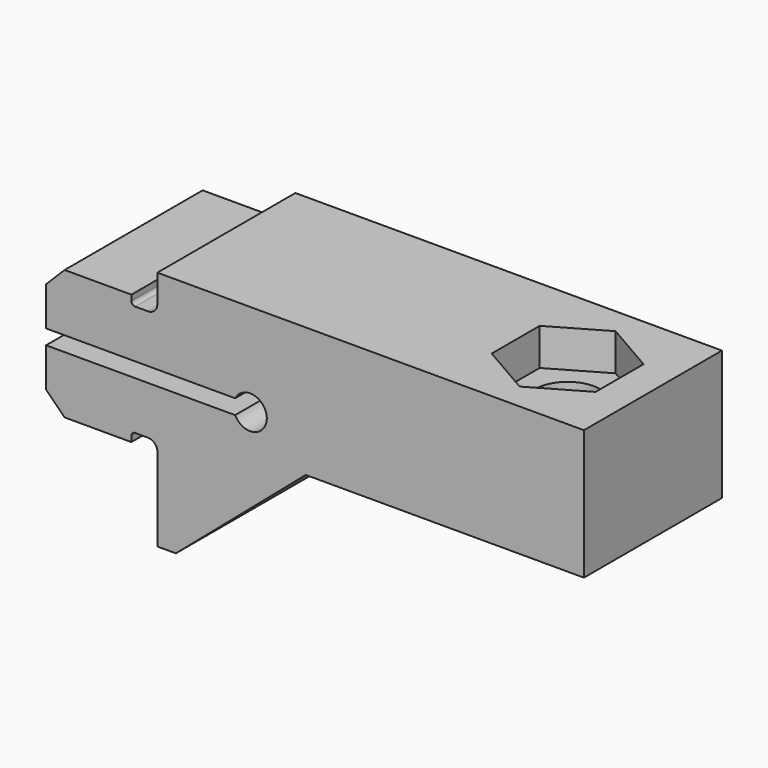
from build123d import *

# Parameters (mm, degrees)
F1_DEPTH = 4.65
F2_R     = 1.75
F3_DEPTH = 13.001
F4_DEPTH = 2
F8_DEPTH = 12.5
F9_SIZE  = 0.99999
F10_R    = 0.5
F11_R    = 0.2
F12_W    = 7
F12_H    = 1.5


# Not quite as in the source:
# - a fillet or chamfer is up to 0.001 mm smaller than in the source, because OpenCascade refuses the exact size


with BuildPart() as f1:
    # F0 (on Front) → F1 (new body, symmetric)
    with BuildSketch(Plane.XZ):
        Polygon((23, 0), (0, 0), (0, -1.5), (0, -2), (-1.4, -2), (-1.4, -1.5), (-6, -1.5), (-6, -8.5), (-1.4, -8.5), (-1.4, -8), (0, -8), (0, -8.5), (0, -13), (1, -13), (8, -7), (23, -7), align=None)
    extrude(amount=F1_DEPTH, both=True)

    # F2 (on face) → F3 (cut, through all)
    with BuildSketch(Plane.XY):
        with Locations((18.4, 0)):
            Circle(F2_R)
    extrude(amount=-F3_DEPTH, mode=Mode.SUBTRACT)

    # F2 (on face) → F4 (cut)
    with BuildSketch(Plane.XY):
        Polygon((18.4, 3.2331615075), (15.6, 1.6165807537), (15.6, -1.6165807537), (18.4, -3.2331615075), (21.2, -1.6165807537), (21.2, 1.6165807537), align=None)
        with Locations((18.4, 0)):
            Circle(F2_R, mode=Mode.SUBTRACT)
    extrude(amount=-F4_DEPTH, mode=Mode.SUBTRACT)

    # F5 (on Front) → F6 (revolve, cut)
    with BuildSketch(Plane.XZ):
        Polygon((-6, -2.5), (-6, -5), (14, -5), (12.9, -3.9), (-4.6, -3.9), align=None)
    revolve(axis=Axis((22.399994296, 0, -5), (1, 0, 0)), mode=Mode.SUBTRACT)

    # F7 (on Front) → F8 (cut, symmetric)
    with BuildSketch(Plane.XZ):
        with BuildLine():
            ThreePointArc((4.1937742252, -5.4), (5.2054224947, -5.8762428879), (5.9, -5))
            ThreePointArc((5.9, -5), (5.2054224947, -4.1237571121), (4.1937742252, -4.6))
            ThreePointArc((4.1937742252, -4.6), (4.1, -5), (4.1937742252, -5.4))
        make_face()
        with BuildLine():
            ThreePointArc((4.1937742252, -5.4), (4.1, -5), (4.1937742252, -4.6))
            Line((4.1937742252, -4.6), (-6, -4.6))
            Line((-6, -4.6), (-6, -5.4))
            Line((-6, -5.4), (4.1937742252, -5.4))
        make_face()
    extrude(amount=F8_DEPTH, both=True, mode=Mode.SUBTRACT)

    # F9 (size 1 in the source; OpenCascade refuses exactly that, so slightly less here)
    f9_edges = [f1.edges().sort_by_distance(p)[0] for p in [
        (-6, 0, -8.5),
        (-6, 0, -1.5),
    ]]
    chamfer(f9_edges, length=F9_SIZE)

    # F10
    f10_edges = [f1.edges().sort_by_distance(p)[0] for p in [
        (0, 0, -2),
        (0, 0, -8),
    ]]
    fillet(f10_edges, radius=F10_R)

    # F11
    f11_edges = [f1.edges().sort_by_distance(p)[0] for p in [
        (-1.4, 0, -2),
        (-1.4, 0, -8),
    ]]
    fillet(f11_edges, radius=F11_R)

    # F12 (on Front) → F13 (revolve, cut)
    with BuildSketch(Plane.XZ):
        with Locations((-2.5, -4.25)):
            Rectangle(F12_W, F12_H)
    revolve(axis=Axis((4, 0, -5), (1, 0, 0)), mode=Mode.SUBTRACT)


solid = f1.part
